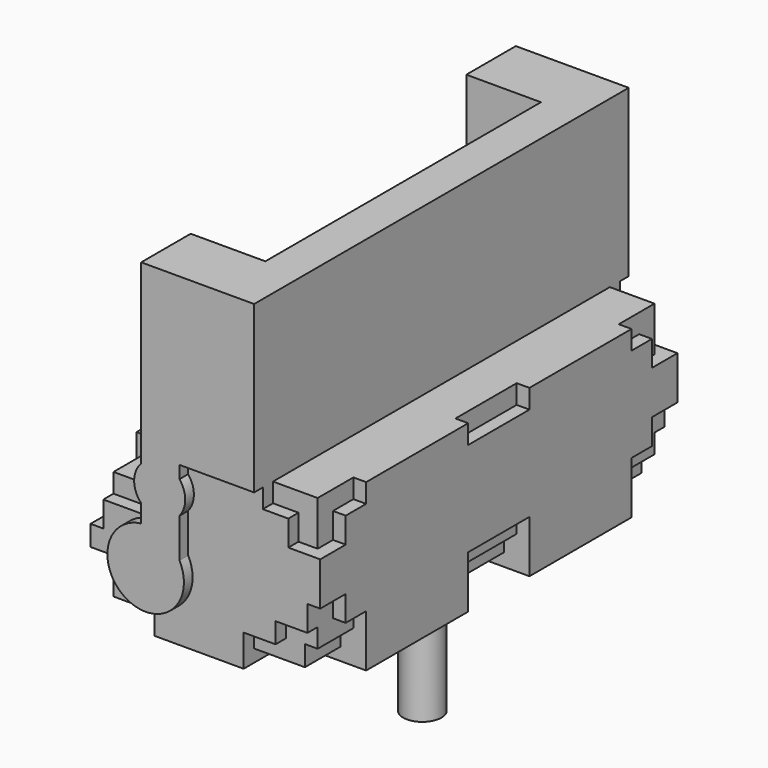
from build123d import *

# Parameters (mm, degrees)
F0_R          = 3
F0_R_2        = 2
F1_DEPTH      = 16.5
F1_DEPTH_BACK = 16.5
F3_DEPTH      = 18.35
F4_DEPTH      = 11
F5_DEPTH      = 18.35
F6_DEPTH      = 18.35
F7_START      = -12
F2_W          = 3
F2_H          = 1.85
F7_DEPTH      = 13
F9_DEPTH      = 1
F11_DEPTH     = 1
F12_W         = 3
F12_H         = 1.85
F12_W_2       = 2.85
F12_W_3       = 4.2
F12_H_2       = 1.5
F13_DEPTH     = 13
F14_DEPTH     = 13
F15_DEPTH     = 8
F16_DEPTH     = 8
F17_W         = 3.3
F17_H         = 10
F18_DEPTH     = 1
F19_W         = 10
F19_H         = 4.4
F20_DEPTH     = 1
F22_DEPTH     = 1.6
F24_DEPTH     = 1
F26_DEPTH     = 1
F28_DEPTH     = 1


with BuildPart() as f1:
    # F0 (on Front) → F1 (new body, two sides)
    with BuildSketch(Plane.XZ) as f1_sk:
        Polygon((0, 8.6), (0, 0), (15, 0), (15, 1.6), (16, 1.6), (16, 12), (2.3, 12), (2.3, 8.6), align=None)
        with Locations((4, 4)):
            Circle(F0_R, mode=Mode.SUBTRACT)
        with Locations((5.1, 9.75)):
            Circle(F0_R_2, mode=Mode.SUBTRACT)
        with Locations((4, 4)):
            Circle(F0_R)
        with Locations((5.1, 9.75)):
            Circle(F0_R_2)
    extrude(amount=F1_DEPTH)
    extrude(f1_sk.sketch, amount=-F1_DEPTH_BACK)

    # F0 (on Front) → F3 (join, symmetric)
    with BuildSketch(Plane.XZ):
        with Locations((4, 4)):
            Circle(F0_R)
    extrude(amount=F3_DEPTH, both=True)

    # F2 (on face) → F4 (join)
    with BuildSketch(Plane(origin=(0, 0, 0), x_dir=(1, 0, 0), z_dir=(0, 0, -1))):
        with BuildLine():
            ThreePointArc((9.5, 0), (11, -1.5), (12.5, 0))
            ThreePointArc((12.5, 0), (11, 1.5), (9.5, 0))
        make_face()
    extrude(amount=F4_DEPTH)

    # F0 (on Front) → F5 (join)
    with BuildSketch(Plane.XZ):
        with Locations((5.1, 9.75)):
            Circle(F0_R_2)
    extrude(amount=F5_DEPTH)

    # F2 (on face) → F7 (join)
    with BuildSketch(Plane(origin=(0, 0, 0), x_dir=(1, 0, 0), z_dir=(0, 0, -1)).offset(F7_START)):
        with Locations((11, 17.425)):
            Rectangle(F2_W, F2_H)
        with BuildLine():
            ThreePointArc((9.5, 2), (11, 2.5), (12.5, 2))
            Line((12.5, 2), (12.5, 16.5))
            Line((12.5, 16.5), (9.5, 16.5))
            Line((9.5, 16.5), (9.5, 2))
        make_face()
        with BuildLine():
            Line((12.5, 0), (12.5, 2))
            ThreePointArc((12.5, 2), (11, 2.5), (9.5, 2))
            Line((9.5, 2), (9.5, 0))
            ThreePointArc((9.5, 0), (11, 1.5), (12.5, 0))
        make_face()
        with BuildLine():
            ThreePointArc((9.5, 0), (11, -1.5), (12.5, 0))
            ThreePointArc((12.5, 0), (11, 1.5), (9.5, 0))
        make_face()
        with BuildLine():
            ThreePointArc((9.5, -2), (11, -2.5), (12.5, -2))
            Line((12.5, -2), (12.5, 0))
            ThreePointArc((12.5, 0), (11, -1.5), (9.5, 0))
            Line((9.5, 0), (9.5, -2))
        make_face()
        with BuildLine():
            Line((12.5, -16.5), (12.5, -2))
            ThreePointArc((12.5, -2), (11, -2.5), (9.5, -2))
            Line((9.5, -2), (9.5, -16.5))
            Line((9.5, -16.5), (12.5, -16.5))
        make_face()
        with Locations((11, -17.425)):
            Rectangle(F2_W, F2_H)
    extrude(amount=-F7_DEPTH)

    # F8 (on face) → F9 (join)
    with BuildSketch(Plane.YZ.offset(16)):
        Polygon((-13, 3.1), (-13, 1.6), (-3, 1.6), (-3, 3.1), (3, 3.1), (3, 1.6), (13, 1.6), (13, 3.1), (15, 3.1), (15, 5.1), (16.5, 5.1), (16.5, 8.5), (15, 8.5), (15, 10.5), (13, 10.5), (13, 12), (3, 12), (3, 10.5), (-3, 10.5), (-3, 12), (-13, 12), (-13, 10.5), (-15, 10.5), (-15, 8.5), (-16.5, 8.5), (-16.5, 5.1), (-15, 5.1), (-15, 3.1), align=None)
    extrude(amount=F9_DEPTH)

    # F10 (on face) → F11 (join)
    with BuildSketch(Plane(origin=(0, 0, 0), x_dir=(0, -1, 0), z_dir=(-1, 0, 0))):
        Polygon((-13, 1.5), (-13, 0), (-3, 0), (-3, 1.5), (3, 1.5), (3, 0), (13, 0), (13, 1.5), (15, 1.5), (15, 3.5), (16.5, 3.5), (16.5, 5.1), (15, 5.1), (15, 7.1), (13, 7.1), (13, 8.6), (3, 8.6), (3, 7.1), (-3, 7.1), (-3, 8.6), (-13, 8.6), (-13, 7.1), (-15, 7.1), (-15, 5.1), (-16.5, 5.1), (-16.5, 3.5), (-15, 3.5), (-15, 1.5), align=None)
    extrude(amount=F11_DEPTH)

    # F12 (on face) → F13 (join, through all)
    with BuildSketch(Plane.XY.offset(12)):
        with Locations((5.15, -17.425)):
            Rectangle(F12_W, F12_H)
        Polygon((6.65, -16.5), (9.5, -16.5), (9.5, -13.5), (8, -13.5), (8, -15), (3.8, -15), (3.8, -13.5), (3.65, -13.5), (3.65, -16.5), align=None)
        with Locations((8.075, -17.425)):
            Rectangle(F12_W_2, F12_H)
        with Locations((5.9, -14.25)):
            Rectangle(F12_W_3, F12_H_2)
    extrude(amount=F13_DEPTH)

    # F12 (on face) → F14 (join, through all)
    with BuildSketch(Plane.XY.offset(12)):
        with Locations((8.075, 17.425)):
            Rectangle(F12_W_2, F12_H)
        with Locations((5.15, 17.425)):
            Rectangle(F12_W, F12_H)
        Polygon((8, 13.5), (9.5, 13.5), (9.5, 16.5), (6.65, 16.5), (3.65, 16.5), (3.65, 13.5), (3.8, 13.5), (3.8, 15), (8, 15), align=None)
        with Locations((5.9, 14.25)):
            Rectangle(F12_W_3, F12_H_2)
    extrude(amount=F14_DEPTH)

    # F12 (on face) → F15 (join)
    with BuildSketch(Plane.XY.offset(12)):
        with Locations((5.15, -17.425)):
            Rectangle(F12_W, F12_H)
    extrude(amount=-F15_DEPTH)

    # F12 (on face) → F16 (join)
    with BuildSketch(Plane.XY.offset(12)):
        with Locations((5.15, 17.425)):
            Rectangle(F12_W, F12_H)
    extrude(amount=-F16_DEPTH)

    # F17 (on face) → F18 (join)
    with BuildSketch(Plane.XY.offset(8.6)):
        with Locations((0.65, -8)):
            Rectangle(F17_W, F17_H)
        with Locations((0.65, 8)):
            Rectangle(F17_W, F17_H)
    extrude(amount=F18_DEPTH)

    # F19 (on face) → F20 (join)
    with BuildSketch(Plane(origin=(2.3, 0, 0), x_dir=(0, -1, 0), z_dir=(-1, 0, 0))):
        with Locations((8, 10.8)):
            Rectangle(F19_W, F19_H)
        with Locations((-8, 10.8)):
            Rectangle(F19_W, F19_H)
    extrude(amount=F20_DEPTH)

    # F21 (on face) → F22 (join, through all)
    with BuildSketch(Plane(origin=(0, 0, 1.6), x_dir=(1, 0, 0), z_dir=(0, 0, -1))):
        Polygon((16, 13), (15, 13), (15, 3), (16, 3), (17, 3), (17, 13), align=None)
        Polygon((16, -3), (15, -3), (15, -13), (16, -13), (17, -13), (17, -3), align=None)
    extrude(amount=F22_DEPTH)

    # F23 (on face) → F24 (join)
    with BuildSketch(Plane(origin=(0, 0, 0), x_dir=(1, 0, 0), z_dir=(0, 0, -1))):
        with BuildLine():
            Line((15, -13), (17, -13))
            Line((17, -13), (17, -3))
            Line((17, -3), (15, -3))
            Line((15, -3), (11.9604686356, -3))
            ThreePointArc((11.9604686356, -3), (7.85, 0), (11.9604686356, 3))
            Line((11.9604686356, 3), (15, 3))
            Line((15, 3), (17, 3))
            Line((17, 3), (17, 13))
            Line((17, 13), (15, 13))
            Line((15, 13), (13.5, 13))
            Line((13.5, 13), (13.5, 15))
            Line((13.5, 15), (11, 15))
            Line((11, 15), (11, 16.5))
            Line((11, 16.5), (4, 16.5))
            Line((4, 16.5), (4, 15))
            Line((4, 15), (1.5, 15))
            Line((1.5, 15), (1.5, 13))
            Line((1.5, 13), (0, 13))
            Line((0, 13), (-1, 13))
            Line((-1, 13), (-1, 3))
            Line((-1, 3), (0, 3))
            Line((0, 3), (1.5, 3))
            Line((1.5, 3), (1.5, -3))
            Line((1.5, -3), (0, -3))
            Line((0, -3), (-1, -3))
            Line((-1, -3), (-1, -13))
            Line((-1, -13), (0, -13))
            Line((0, -13), (1.5, -13))
            Line((1.5, -13), (1.5, -15))
            Line((1.5, -15), (4, -15))
            Line((4, -15), (4, -16.5))
            Line((4, -16.5), (9.4604686356, -16.5))
            Line((9.4604686356, -16.5), (9.4604686356, -15))
            Line((9.4604686356, -15), (11.9604686356, -15))
            Line((11.9604686356, -15), (11.9604686356, -13))
            Line((11.9604686356, -13), (15, -13))
        make_face()
    extrude(amount=F24_DEPTH)

    # F25 (on face) → F26 (join)
    with BuildSketch(Plane(origin=(0, 16.5, 0), x_dir=(-1, 0, 0), z_dir=(0, 1, 0))):
        with BuildLine():
            Line((-12.5, 10.5), (-14.5, 10.5))
            Line((-14.5, 10.5), (-14.5, 8.5))
            Line((-14.5, 8.5), (-16, 8.5))
            Line((-16, 8.5), (-17, 8.5))
            Line((-17, 8.5), (-17, 5.1))
            Line((-17, 5.1), (-16, 5.1))
            Line((-16, 5.1), (-16, 3.1))
            Line((-16, 3.1), (-13.5, 3.1))
            Line((-13.5, 3.1), (-13.5, 1.5))
            Line((-13.5, 1.5), (-9.4604686356, 1.5))
            Line((-9.4604686356, 1.5), (-9.4604686356, 0))
            Line((-9.4604686356, 0), (-9.4604686356, -1))
            Line((-9.4604686356, -1), (-4, -1))
            Line((-4, -1), (-4, 0))
            Line((-4, 0), (-4, 1))
            ThreePointArc((-4, 1), (-6.5708664233, 2.4538286533), (-6.65, 5.406236111))
            Line((-6.65, 5.406236111), (-6.65, 12))
            Line((-6.65, 12), (-12.5, 12))
            Line((-12.5, 12), (-12.5, 10.5))
        make_face()
    extrude(amount=F26_DEPTH)

    # F27 (on face) → F28 (join)
    with BuildSketch(Plane.XZ.offset(16.5)):
        with BuildLine():
            Line((4, 0), (4, -1))
            Line((4, -1), (11, -1))
            Line((11, -1), (11, 0))
            Line((11, 0), (11, 1.5))
            Line((11, 1.5), (13.5, 1.5))
            Line((13.5, 1.5), (13.5, 3.1))
            Line((13.5, 3.1), (16, 3.1))
            Line((16, 3.1), (16, 5.1))
            Line((16, 5.1), (17, 5.1))
            Line((17, 5.1), (17, 8.5))
            Line((17, 8.5), (16, 8.5))
            Line((16, 8.5), (14.5, 8.5))
            Line((14.5, 8.5), (14.5, 10.5))
            Line((14.5, 10.5), (12.5, 10.5))
            Line((12.5, 10.5), (12.5, 12))
            Line((12.5, 12), (6.65, 12))
            Line((6.65, 12), (6.65, 11.013922466))
            ThreePointArc((6.65, 11.013922466), (7.1, 9.75), (6.65, 8.486077534))
            Line((6.65, 8.486077534), (6.65, 5.406236111))
            ThreePointArc((6.65, 5.406236111), (6.5708664233, 2.4538286533), (4, 1))
            Line((4, 1), (4, 0))
        make_face()
        with BuildLine():
            Line((-1, 3.5), (0, 3.5))
            Line((0, 3.5), (1.0419601085, 3.5))
            ThreePointArc((1.0419601085, 3.5), (1.599471865, 5.7992956047), (3.65, 6.9795133831))
            Line((3.65, 6.9795133831), (3.65, 7.1))
            Line((3.65, 7.1), (0, 7.1))
            Line((0, 7.1), (0, 5.1))
            Line((0, 5.1), (-1, 5.1))
            Line((-1, 5.1), (-1, 3.5))
        make_face()
    extrude(amount=F28_DEPTH)


with BuildPart() as f6:
    # F0 (on Front) → F6 (new body)
    with BuildSketch(Plane.XZ):
        with Locations((5.1, 9.75)):
            Circle(F0_R_2)
    extrude(amount=-F6_DEPTH)


solid = Compound([f1.part, f6.part])
